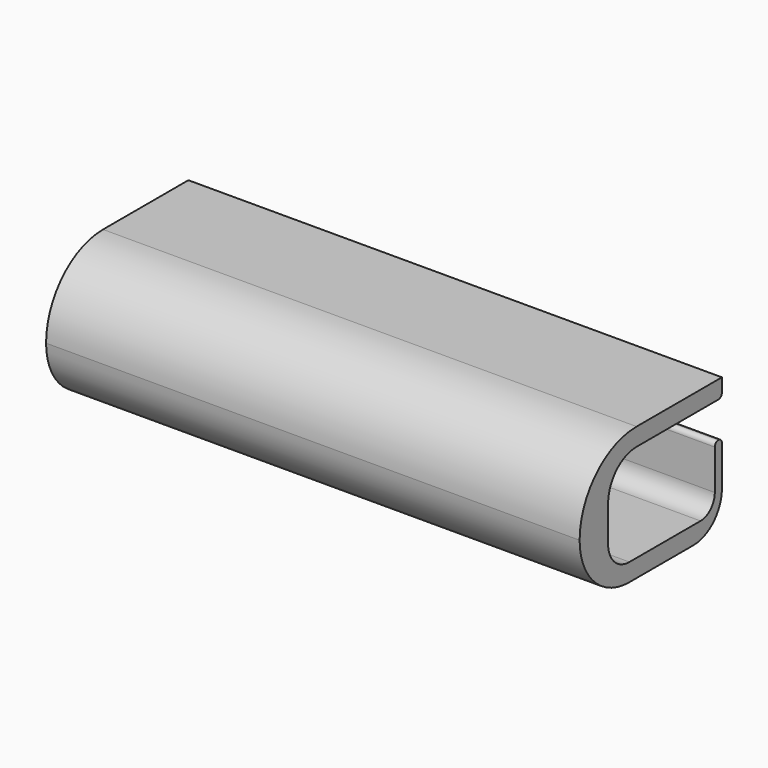
from build123d import *

# Parameters (mm, degrees)
F1_DEPTH = 300
F2_R     = 2.49999


# Not quite as in the source:
# - a fillet or chamfer is up to 0.001 mm smaller than in the source, because OpenCascade refuses the exact size


with BuildPart() as f1:
    # F0 (on Right) → F1 (new body)
    with BuildSketch(Plane.YZ):
        with BuildLine():
            Line((0, -10), (0, 0))
            Line((0, 0), (-60, 0))
            ThreePointArc((-60, 0), (-88.2842712475, -11.7157287525), (-100, -40))
            ThreePointArc((-100, -40), (-89.7487373415, -64.7487373415), (-65, -75))
            Line((-65, -75), (-20, -75))
            ThreePointArc((-20, -75), (-5.8578643763, -69.1421356237), (0, -55))
            Line((0, -55), (0, -30))
            Line((0, -30), (-5, -30))
            Line((-5, -30), (-5, -55))
            ThreePointArc((-5, -55), (-7.9289321881, -62.0710678119), (-15, -65))
            Line((-15, -65), (-65, -65))
            ThreePointArc((-65, -65), (-75.6066017178, -60.6066017178), (-80, -50))
            Line((-80, -50), (-80, -30))
            ThreePointArc((-80, -30), (-74.1421356237, -15.8578643763), (-60, -10))
            Line((-60, -10), (0, -10))
        make_face()
    extrude(amount=F1_DEPTH)

    # F2 (radius 2.5 in the source; OpenCascade refuses exactly that, so slightly less here)
    f2_edges = [f1.edges().sort_by_distance(p)[0] for p in [
        (150, 0, -10),
        (150, 0, -30),
        (150, -5, -30),
    ]]
    fillet(f2_edges, radius=F2_R)


solid = f1.part
